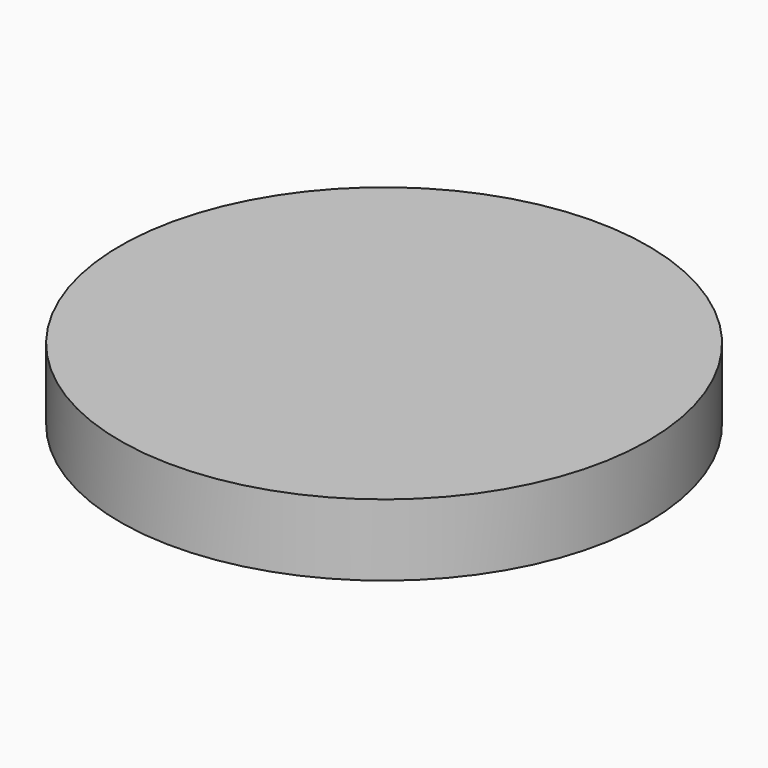
from build123d import *

# Parameters (mm, degrees)
F0_R     = 20.5
F0_R_2   = 13.65
F1_DEPTH = 1.5
F5_COUNT = 13
F6_R     = 20.5
F7_DEPTH = 2.778125


with BuildPart() as f1:
    # F0 (on Top) → F1 (new body, symmetric)
    with BuildSketch(Plane.XY):
        Circle(F0_R)
        Circle(F0_R_2, mode=Mode.SUBTRACT)
    extrude(amount=F1_DEPTH, both=True)



with BuildPart() as f3:
    # F2 (on Top) → F3 (revolve)
    with BuildSketch(Plane.XY):
        with BuildLine():
            Line((-19.853125, 0), (-14.296875, 0))
            ThreePointArc((-14.296875, 0), (-17.075, 2.778125), (-19.853125, 0))
        make_face()
    revolve(axis=Axis((-17.075, 0, 0), (1, 0, 0)))


with BuildPart() as f1_1:
    add(f1.part)

    add(f3.part)  # F5 merges F3
    # F5: F3 ×13 about axis
    f5_axis = Axis((0, 0, 23.2233777642), (0, 0, 1))
    for i in range(1, F5_COUNT):
        add(f3.part.rotate(f5_axis, i * 360 / F5_COUNT))


with BuildPart() as f7:
    # F6 (on Top) → F7 (new body, symmetric)
    with BuildSketch(Plane.XY):
        Circle(F6_R)
    extrude(amount=F7_DEPTH, both=True)


solid = Compound([f1_1.part, f7.part])
